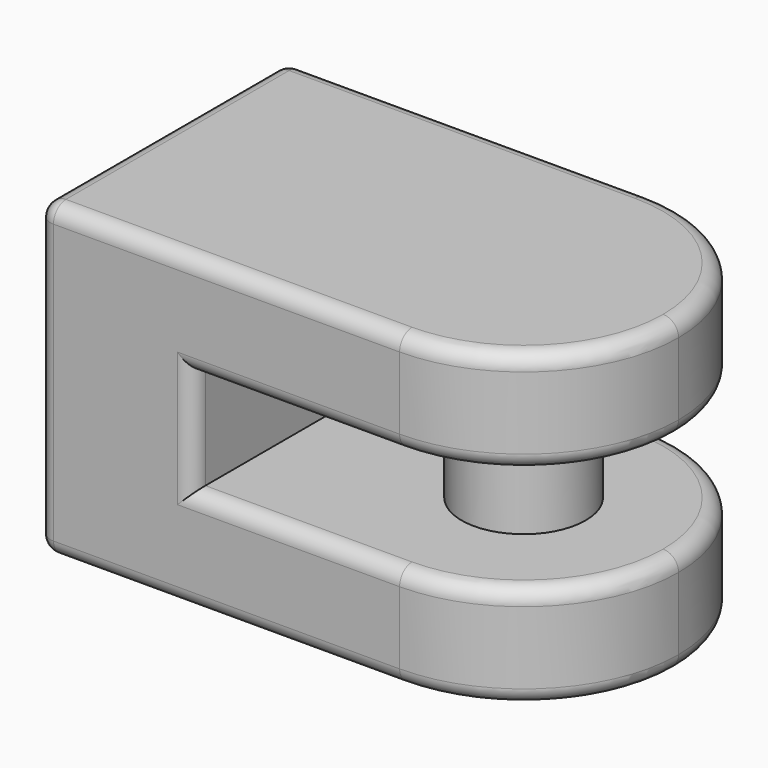
from build123d import *

# Parameters (mm, degrees)
F1_DEPTH = 5.08
F2_R     = 3.048
F3_DEPTH = 5.08
F5_DEPTH = 5.08
F6_W     = 7.62
F6_H     = 15.24
F7_DEPTH = 5.08
F8_R     = 0.762


# Not quite as in the source:
# - a feature names something its author has since deleted; it is built from what else it names


with BuildPart() as f1:
    # F0 (on Top) → F1 (new body)
    with BuildSketch(Plane.XY):
        with BuildLine():
            ThreePointArc((0, -7.62), (-7.62, 0), (0, 7.62))
            Line((0, 7.62), (-17.78, 7.62))
            Line((-17.78, 7.62), (-17.78, -7.62))
            Line((-17.78, -7.62), (0, -7.62))
        make_face()
        with BuildLine():
            Line((0, -7.62), (0, 7.62))
            ThreePointArc((0, 7.62), (-7.62, 0), (0, -7.62))
        make_face()
        with BuildLine():
            ThreePointArc((0, -7.62), (5.3881536726, -5.3881536726), (7.62, 0))
            ThreePointArc((7.62, 0), (5.3881536726, 5.3881536726), (0, 7.62))
            Line((0, 7.62), (0, -7.62))
        make_face()
    extrude(amount=F1_DEPTH)

    # F2 (on face) → F3 (join)
    with BuildSketch(Plane.XY.offset(5.08)):
        Circle(F2_R)
    extrude(amount=F3_DEPTH)

    # F4 (on face) → F5 (join)
    with BuildSketch(Plane.XY.offset(10.16)):
        with BuildLine():
            ThreePointArc((0, -7.62), (5.3881536726, -5.3881536726), (7.62, 0))
            ThreePointArc((7.62, 0), (5.3881536726, 5.3881536726), (0, 7.62))
            Line((0, 7.62), (0, 3.048))
            ThreePointArc((0, 3.048), (2.1552614691, 2.1552614691), (3.048, 0))
            ThreePointArc((3.048, 0), (2.1552614691, -2.1552614691), (0, -3.048))
            Line((0, -3.048), (0, -7.62))
        make_face()
        with BuildLine():
            Line((0, 3.048), (0, 7.62))
            ThreePointArc((0, 7.62), (-7.62, 0), (0, -7.62))
            Line((0, -7.62), (0, -3.048))
            ThreePointArc((0, -3.048), (-3.048, 0), (0, 3.048))
        make_face()
        with BuildLine():
            ThreePointArc((0, -7.62), (-7.62, 0), (0, 7.62))
            Line((0, 7.62), (-17.78, 7.62))
            Line((-17.78, 7.62), (-17.78, -7.62))
            Line((-17.78, -7.62), (0, -7.62))
        make_face()
        with BuildLine():
            ThreePointArc((0, -7.62), (5.3881536726, -5.3881536726), (7.62, 0))
            ThreePointArc((7.62, 0), (5.3881536726, 5.3881536726), (0, 7.62))
            Line((0, 7.62), (0, -7.62))
        make_face()
        with BuildLine():
            Line((0, -7.62), (0, 7.62))
            ThreePointArc((0, 7.62), (-7.62, 0), (0, -7.62))
        make_face()
    extrude(amount=F5_DEPTH)

    # F6 (on face) → F7 (join)
    with BuildSketch(Plane.XY.offset(5.08)):
        with Locations((-13.97, 0)):
            Rectangle(F6_W, F6_H)
    extrude(amount=F7_DEPTH)

    # F8
    f8_edges = [f1.edges().sort_by_distance(p)[0] for p in [
        (-8.89, 7.62, 0),
        (7.62, 0, 0),
        (-8.89, -7.62, 0),
        (7.62, 0, 15.24),
        (-17.78, 7.62, 7.62),
        (-17.78, 0, 0),
        (-17.78, -7.62, 7.62),
        (-17.78, 0, 15.24),
        (7.62, 0, 5.08),
        (7.62, 0, 10.16),
        (-10.16, -7.62, 7.62),
        (-10.16, 7.62, 7.62),
        (-8.89, 7.62, 15.24),
        (-8.89, -7.62, 15.24),
        (-5.08, -7.62, 5.08),
        (-5.08, 7.62, 5.08),
        (-5.08, -7.62, 10.16),
        (-5.08, 7.62, 10.16),
    ]]
    fillet(f8_edges, radius=F8_R)


solid = f1.part
